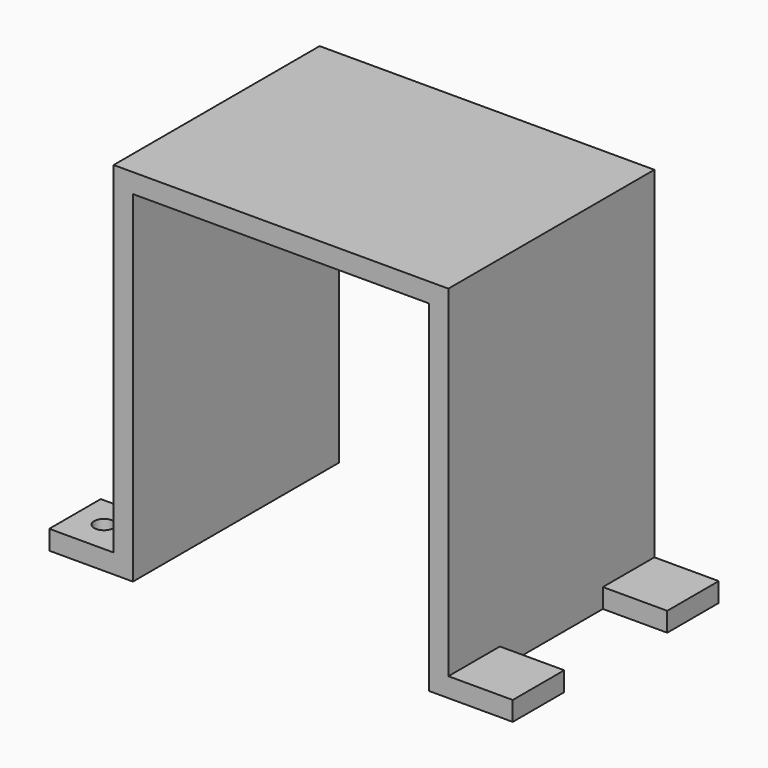
from build123d import *

# Parameters (mm, degrees)
F1_DEPTH = 40
F3_W     = 10
F3_H     = 10
F4_DEPTH = 3
F2_W     = 10
F2_H     = 10
F5_DEPTH = 3
F6_W     = 10
F6_H     = 10
F7_DEPTH = 3
F8_W     = 10
F8_H     = 10
F9_DEPTH = 3
F11_D    = 3


# Not quite as in the source:
# - a feature of the source that left no trace in its solid (it failed there, or was rolled back) is left out
# - a feature names something its author has since deleted; it is built from what else it names


with BuildPart() as f1:
    # F0 (on Front) → F1 (new body)
    with BuildSketch(Plane.XZ):
        Polygon((-56.1606403851, 0), (-56.1606403851, -56), (-53.1606403851, -56), (-53.1606403851, -3), (-7.1606403851, -3), (-7.1606403851, -56), (-4.1606403851, -56), (-4.1606403851, 0), align=None)
    extrude(amount=F1_DEPTH)

    # F3 (on face) → F4 (join)
    with BuildSketch(Plane(origin=(0, 0, -56), x_dir=(1, 0, 0), z_dir=(0, 0, -1))):
        with Locations((0.8393596149, 5)):
            Rectangle(F3_W, F3_H)
    extrude(amount=-F4_DEPTH)

    # F2 (on face) → F5 (join)
    with BuildSketch(Plane(origin=(0, 0, -56), x_dir=(1, 0, 0), z_dir=(0, 0, -1))):
        with Locations((-61.1606403851, 5)):
            Rectangle(F2_W, F2_H)
    extrude(amount=-F5_DEPTH)

    # F6 (on face) → F7 (join)
    with BuildSketch(Plane(origin=(0, 0, -56), x_dir=(1, 0, 0), z_dir=(0, 0, -1))):
        with Locations((0.8393596149, 35)):
            Rectangle(F6_W, F6_H)
    extrude(amount=-F7_DEPTH)

    # F8 (on face) → F9 (join)
    with BuildSketch(Plane(origin=(0, 0, -56), x_dir=(1, 0, 0), z_dir=(0, 0, -1))):
        with Locations((-61.1606403851, 35)):
            Rectangle(F8_W, F8_H)
    extrude(amount=-F9_DEPTH)

    # F11 (through all)
    with Locations(Plane(origin=(0, 0, -56), x_dir=(1, 0, 0), z_dir=(0, 0, -1))):
        with Locations((-61.6680905223, 35), (18.8430529088, 95.1308980584), (-61.3079555333, 4.5014377683), (19.3945541978, 4.6852682717)):
            Hole(F11_D / 2)


solid = f1.part
